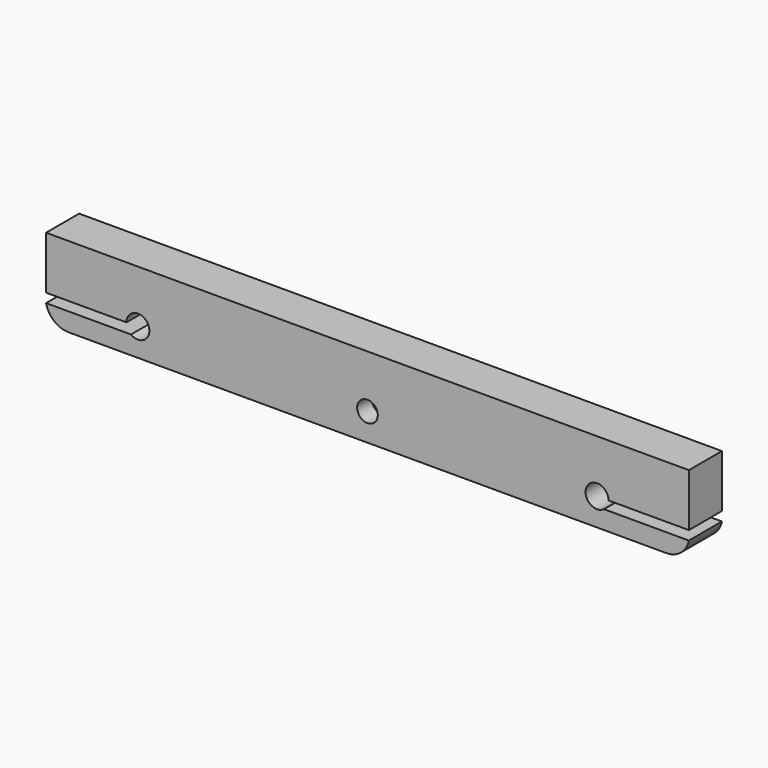
from build123d import *

# Parameters (mm, degrees)
F0_R        = 11
F0_R_2      = 4.5
F1_DEPTH    = 18
F2_DEPTH    = 10
F3_T1_DEPTH = 66.9897948557


# Not quite as in the source:
# - a fillet or chamfer that OpenCascade refuses, or shapes differently, is made with other operations: its cross-section is extruded or revolved along the edge and cut away or added
# - a feature names something its author has since deleted; it is built from what else it names


with BuildPart() as f1:
    # F0 (on Front) → F1 (new body)
    with BuildSketch(Plane.XZ):
        with BuildLine():
            Line((-47.1908605099, -35.0622619203), (-327.1908605099, -35.0622619203))
            Line((-327.1908605099, -35.0622619203), (-327.1908605099, -58.0622619203))
            Line((-327.1908605099, -58.0622619203), (-292.1908605099, -58.0622619203))
            ThreePointArc((-292.1908605099, -58.0622619203), (-287.1908605099, -53.0622619203), (-282.1908605099, -58.0622619203))
            ThreePointArc((-282.1908605099, -58.0622619203), (-284.9547925324, -62.5343978753), (-290.1908605099, -62.0622619203))
            Line((-290.1908605099, -62.0622619203), (-327.1908605099, -62.0622619203))
            Line((-327.1908605099, -62.0622619203), (-327.1908605099, -70.0622619203))
            Line((-327.1908605099, -70.0622619203), (-47.1908605099, -70.0622619203))
            Line((-47.1908605099, -70.0622619203), (-47.1908605099, -62.0622619203))
            Line((-47.1908605099, -62.0622619203), (-84.1908605099, -62.0622619203))
            ThreePointArc((-84.1908605099, -62.0622619203), (-91.6629964649, -55.8261939428), (-82.1908605099, -58.0622619203))
            Line((-82.1908605099, -58.0622619203), (-47.1908605099, -58.0622619203))
            Line((-47.1908605099, -58.0622619203), (-47.1908605099, -35.0622619203))
        make_face()
        with Locations((-187.1908605099, -58.0622619203)):
            Circle(F0_R, mode=Mode.SUBTRACT)
        with Locations((-187.1908605099, -58.0622619203)):
            Circle(F0_R)
        with Locations((-187.1908605099, -58.0622619203)):
            Circle(F0_R_2, mode=Mode.SUBTRACT)
    extrude(amount=F1_DEPTH)

    # F0 (on Front) → F2 (cut)
    with BuildSketch(Plane.XZ):
        with Locations((-187.1908605099, -58.0622619203)):
            Circle(F0_R)
        with Locations((-187.1908605099, -58.0622619203)):
            Circle(F0_R_2, mode=Mode.SUBTRACT)
    extrude(amount=F2_DEPTH, mode=Mode.SUBTRACT)

    # F3: fillet of radius 10 on 2 edges, made by hand

    # F3_s2 → F3_t1 (cut)
    with BuildSketch(Plane.XZ.offset(-24.4948974278)):
        with BuildLine():
            ThreePointArc((-317.3929015387, -70.0622619203), (-323.7174568591, -67.8082286127), (-327.1908605099, -62.0622619203))
            Line((-327.1908605099, -62.0622619203), (-327.1908605099, -70.0622619203))
            Line((-327.1908605099, -70.0622619203), (-317.3929015387, -70.0622619203))
        make_face()
        with BuildLine():
            ThreePointArc((-47.1908605099, -62.0622619203), (-50.6642641607, -67.8082286127), (-56.988819481, -70.0622619203))
            Line((-56.988819481, -70.0622619203), (-47.1908605099, -70.0622619203))
            Line((-47.1908605099, -70.0622619203), (-47.1908605099, -62.0622619203))
        make_face()
    extrude(amount=F3_T1_DEPTH, mode=Mode.SUBTRACT)


solid = f1.part
